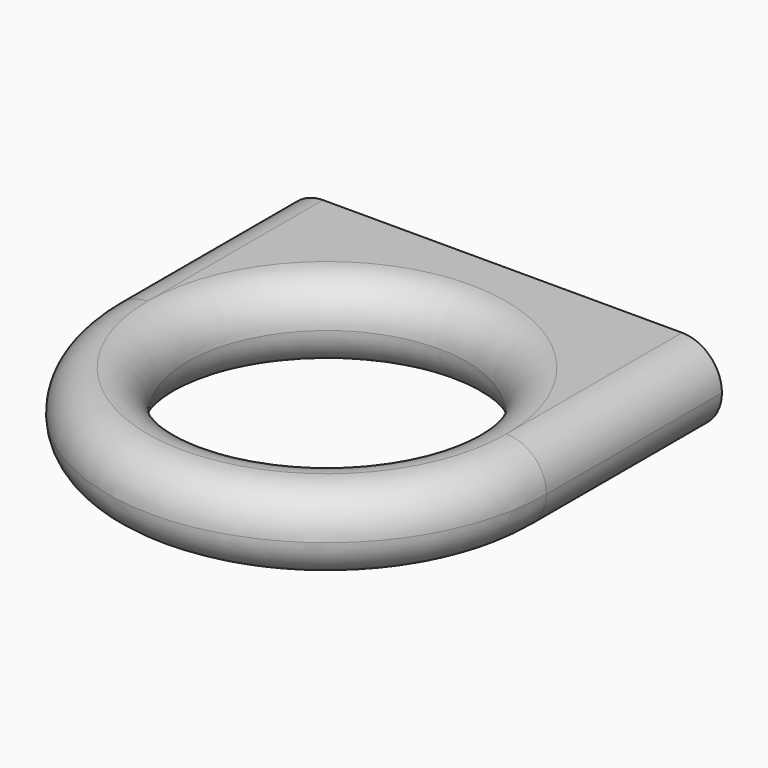
from build123d import *

# Parameters (mm, degrees)
F2_DEPTH = 5
F3_R     = 4.99999
F5_D     = 5
F5_DEPTH = 17.5
F5_TIP   = 1.5021515476
F6_D     = 5
F6_DEPTH = 17.5
F6_TIP   = 1.5021515476


# Not quite as in the source:
# - a fillet or chamfer is up to 0.001 mm smaller than in the source, because OpenCascade refuses the exact size


with BuildPart() as f2:
    # F1 (on Top) → F2 (new body, symmetric)
    with BuildSketch(Plane.XY):
        with BuildLine():
            Line((27.5, 0), (17.5, 0))
            ThreePointArc((17.5, 0), (0, -17.5), (-17.5, 0))
            Line((-17.5, 0), (-27.5, 0))
            ThreePointArc((-27.5, 0), (0, -27.5), (27.5, 0))
        make_face()
        with BuildLine():
            ThreePointArc((-17.5, 0), (0, 17.5), (17.5, 0))
            Line((17.5, 0), (27.5, 0))
            Line((27.5, 0), (27.5, 27.5))
            Line((27.5, 27.5), (0, 27.5))
            Line((0, 27.5), (-27.5, 27.5))
            Line((-27.5, 27.5), (-27.5, 0))
            Line((-27.5, 0), (-17.5, 0))
        make_face()
    extrude(amount=F2_DEPTH, both=True)

    # F3 (radius 5 in the source; OpenCascade refuses exactly that, so slightly less here)
    f3_edges = [f2.edges().sort_by_distance(p)[0] for p in [
        (17.5, 0, -5),
        (0, -27.5, -5),
        (0, -27.5, 5),
        (17.5, 0, 5),
    ]]
    fillet(f3_edges, radius=F3_R)

    # F5
    with Locations(Plane(origin=(0, 27.5, 0), x_dir=(-1, 0, 0), z_dir=(0, 1, 0))):
        with Locations((-22.5, 0)):
            Hole(F5_D / 2, depth=F5_DEPTH)
            with Locations((0, 0, -(F5_DEPTH + F5_TIP / 2))):  # 118° drill point
                Cone(0, F5_D / 2, F5_TIP, mode=Mode.SUBTRACT)

    # F6
    with Locations(Plane(origin=(0, 27.5, 0), x_dir=(-1, 0, 0), z_dir=(0, 1, 0))):
        with Locations((22.5, 0)):
            Hole(F6_D / 2, depth=F6_DEPTH)
            with Locations((0, 0, -(F6_DEPTH + F6_TIP / 2))):  # 118° drill point
                Cone(0, F6_D / 2, F6_TIP, mode=Mode.SUBTRACT)


solid = f2.part
